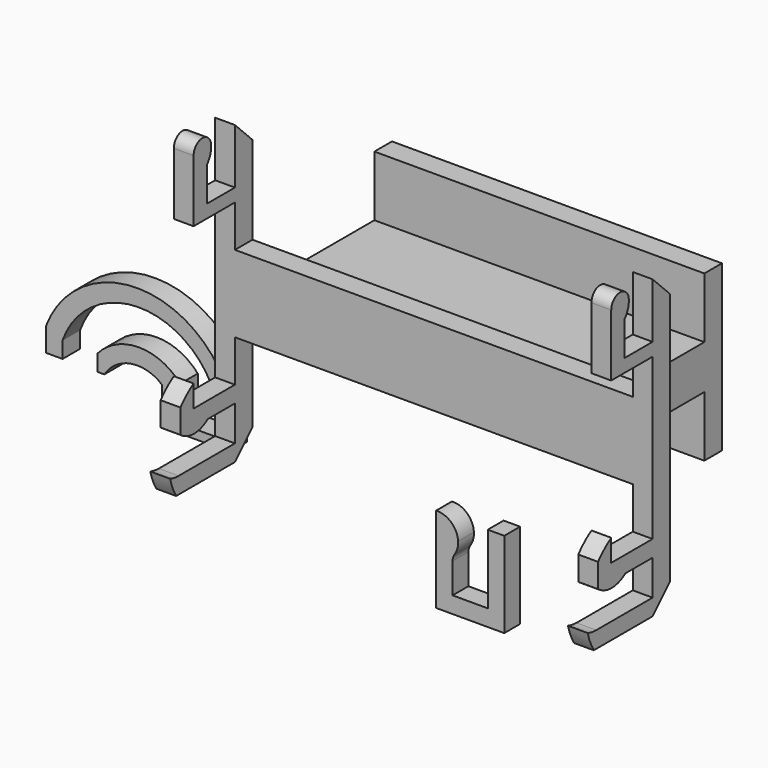
from build123d import *

# Parameters (mm, degrees)
F1_DEPTH  = 5.08
F2_W      = 3.81
F2_H      = 3.81
F2_H_2    = 16.002
F3_DEPTH  = 4.572
F4_R      = 2.54
F6_DEPTH  = 8.89
F5_W      = 12.065
F5_H      = 25.4
F7_W      = 76.2508
F7_H      = 38.1
F8_DEPTH  = 5.08
F11_DEPTH = 50.546
F12_W     = 12.4206
F12_H     = 25.4
F13_DEPTH = 25.4
F14_W     = 91.948
F14_H     = 25.4
F15_DEPTH = 25.4
F16_W     = 8.128
F16_H     = 3.0225940797
F16_W_2   = 3.81
F17_DEPTH = 50.546
F18_R     = 2.54
F19_SIZE  = 5.07999
F20_SIZE  = 5.07999
F22_DEPTH = 25.4
F23_SIZE  = 5.08
F24_SIZE  = 5.08
F25_DEPTH = 57.15
F26_R     = 7.62
F27_R     = 7.62
F29_DEPTH = 101.092


# Not quite as in the source:
# - a fillet or chamfer is up to 0.001 mm smaller than in the source, because OpenCascade refuses the exact size
# - a feature names something its author has since deleted; it is built from what else it names


with BuildPart() as f1:
    # F0 (on Front) → F1 (new body)
    with BuildSketch(Plane.XZ):
        with BuildLine():
            Line((-13.6702175791, 3.3680211509), (-13.6702175791, 11.4960211509))
            ThreePointArc((-13.6702175791, 11.4960211509), (-23.1952175791, 15.7957607383), (-32.7202175791, 11.4960211509))
            Line((-32.7202175791, 11.4960211509), (-32.7202175791, 7.6860211509))
            Line((-32.7202175791, 7.6860211509), (-31.1910058421, 7.6860211509))
            ThreePointArc((-31.1910058421, 7.6860211509), (-25.0379678472, 11.8650180854), (-17.8627536235, 9.9053771004))
            Line((-17.8627536235, 9.9053771004), (-17.8627536235, 1.3360211509))
            Line((-17.8627536235, 1.3360211509), (-2.2494181128, 1.3360211509))
            Line((-2.2494181128, 1.3360211509), (-2.2494181128, 12.5290875188))
            ThreePointArc((-2.2494181128, 12.5290875188), (-23.214575579, 27.7308374634), (-44.6582175791, 13.2118413985))
            Line((-44.6582175791, 13.2118413985), (-44.6582175791, 7.6860211509))
            Line((-44.6582175791, 7.6860211509), (-40.8482175791, 7.6860211509))
            Line((-40.8482175791, 7.6860211509), (-40.8482175791, 11.4960211509))
            ThreePointArc((-40.8482175791, 11.4960211509), (-23.3892785102, 23.9227565337), (-5.6768820684, 11.8600322155))
            Line((-5.6768820684, 11.8600322155), (-5.6768820684, 3.3680211509))
            Line((-5.6768820684, 3.3680211509), (-13.6702175791, 3.3680211509))
        make_face()
    extrude(amount=F1_DEPTH)


with BuildPart() as f3:
    # F2 (on Front) → F3 (new body)
    with BuildSketch(Plane.XZ):
        with Locations((46.9784255706, -13.335)):
            Rectangle(F2_W, F2_H)
        Polygon((60.8214255706, -15.24), (60.8214255706, -11.43), (57.0114255706, -11.43), (48.8834255706, -11.43), (48.8834255706, -15.24), align=None)
        with BuildLine():
            Line((45.0734255706, -11.43), (48.8834255706, -11.43))
            Line((48.8834255706, -11.43), (48.8834255706, -3.556))
            ThreePointArc((48.8834255706, -3.556), (49.8785151524, -1.9066034221), (50.1534255706, 0))
            ThreePointArc((50.1534255706, 0), (48.5549154183, 3.3320998308), (45.0734255706, 4.572))
            Line((45.0734255706, 4.572), (45.0734255706, -11.43))
        make_face()
        with Locations((58.9164255706, -3.429)):
            Rectangle(F2_W, F2_H_2)
    extrude(amount=F3_DEPTH)

    # F4
    f4_edges = [f3.edges().sort_by_distance(p)[0] for p in [
        (48.883426, -2.286, -3.556),
    ]]
    fillet(f4_edges, radius=F4_R)


with BuildPart() as f6:
    # F5 (on Front) → F6 (new body)
    with BuildSketch(Plane.XZ):
        with BuildLine():
            Line((64.2612756615, 64.0052915247), (64.2612756615, 56.3852915247))
            ThreePointArc((64.2612756615, 56.3852915247), (65.1168167537, 54.3198326169), (67.1822756615, 53.4642915247))
            Line((67.1822756615, 53.4642915247), (84.0748242118, 53.4642915247))
            Line((84.0748242118, 53.4642915247), (88.6452756615, 58.0347429745))
            Line((88.6452756615, 58.0347429745), (88.6452756615, 62.3558400749))
            Line((88.6452756615, 62.3558400749), (84.0748242118, 66.9262915247))
            Line((84.0748242118, 66.9262915247), (67.1822756615, 66.9262915247))
            ThreePointArc((67.1822756615, 66.9262915247), (65.1168167537, 66.0707504326), (64.2612756615, 64.0052915247))
        make_face()
        with BuildLine():
            Line((83.5487729875, 54.7342915247), (67.1822756615, 54.7342915247))
            ThreePointArc((67.1822756615, 54.7342915247), (66.0148423658, 55.217858229), (65.5312756615, 56.3852915247))
            Line((65.5312756615, 56.3852915247), (65.5312756615, 64.0052915247))
            ThreePointArc((65.5312756615, 64.0052915247), (66.0148423658, 65.1727248204), (67.1822756615, 65.6562915247))
            Line((67.1822756615, 65.6562915247), (83.5487729875, 65.6562915247))
            Line((83.5487729875, 65.6562915247), (87.3752756615, 61.8297888507))
            Line((87.3752756615, 61.8297888507), (87.3752756615, 58.5607941987))
            Line((87.3752756615, 58.5607941987), (83.5487729875, 54.7342915247))
        make_face(mode=Mode.SUBTRACT)
    extrude(amount=F6_DEPTH)



with BuildPart() as f6b:
    # F5 (on Front) → F6, piece 2 (new body)
    with BuildSketch(Plane.XZ):
        with Locations((53.9104570084, 60.1952915247)):
            Rectangle(F5_W, F5_H)
    extrude(amount=F6_DEPTH)


with BuildPart() as f6c:
    # F5 (on Front) → F6, piece 3 (new body)
    with BuildSketch(Plane.XZ):
        with Locations((98.9955507601, 60.1952915247)):
            Rectangle(F5_W, F5_H)
    extrude(amount=F6_DEPTH)


with BuildPart() as f6_1:
    add(f6.part)

    add(f6b.part)  # F8 merges F6b

    add(f6c.part)  # F8 merges F6c
    # F7 (on face) → F8 (join)
    with BuildSketch(Plane.XZ.offset(8.89)):
        with Locations((76.4530038843, 60.1952915247)):
            Rectangle(F7_W, F7_H)
        Polygon((59.9429570084, 47.4952915247), (47.8779570084, 47.4952915247), (47.8779570084, 72.8952915247), (59.9429570084, 72.8952915247), (59.9429570084, 67.5330780989), (76.4530038843, 60.1952915247), (59.9429570084, 52.8575049505), align=None, mode=Mode.SUBTRACT)
        Polygon((59.9429570084, 72.8952915247), (47.8779570084, 72.8952915247), (59.9429570084, 67.5330780989), align=None)
        Polygon((59.9429570084, 67.5330780989), (59.9429570084, 52.8575049505), (76.4530038843, 60.1952915247), align=None)
        Polygon((47.8779570084, 72.8952915247), (47.8779570084, 47.4952915247), (59.9429570084, 52.8575049505), (59.9429570084, 67.5330780989), align=None)
        Polygon((59.9429570084, 52.8575049505), (47.8779570084, 47.4952915247), (59.9429570084, 47.4952915247), align=None)
    extrude(amount=F8_DEPTH)

    # F10 (on offset) → F11 (join, symmetric)
    with BuildSketch(Plane(origin=(76.4530038843, 0, 0), x_dir=(0, -1, 0), z_dir=(-1, 0, 0))):
        Polygon((39.37, 65.2752915247), (13.97, 65.2752915247), (13.97, 60.1952915247), (44.45, 60.1952915247), (44.45, 94.4852915247), (39.37, 94.4852915247), align=None)
        Polygon((44.45, 60.1952915247), (13.97, 60.1952915247), (13.97, 55.1152915247), (39.37, 55.1152915247), (39.37, 25.9052915247), (44.45, 25.9052915247), align=None)
    extrude(amount=F11_DEPTH, both=True)

    # F12 (on face) → F13 (cut)
    with BuildSketch(Plane.XY.offset(65.2752915247)):
        with Locations((32.1173038843, -26.67)):
            Rectangle(F12_W, F12_H)
        with Locations((120.7887038843, -26.67)):
            Rectangle(F12_W, F12_H)
    extrude(amount=-F13_DEPTH, mode=Mode.SUBTRACT)

    # F14 (on face) → F15 (cut)
    with BuildSketch(Plane.XZ.offset(44.45)):
        with Locations((76.4530038843, 81.7852915247)):
            Rectangle(F14_W, F14_H)
        with Locations((76.4530038843, 38.6052915247)):
            Rectangle(F14_W, F14_H)
    extrude(amount=-F15_DEPTH, mode=Mode.SUBTRACT)

    # F16 (on offset) → F17 (join, symmetric)
    with BuildSketch(Plane(origin=(76.4530038843, 0, 0), x_dir=(0, -1, 0), z_dir=(-1, 0, 0))):
        with Locations((48.514, 80.2485885645)):
            Rectangle(F16_W, F16_H)
        Polygon((68.326, 29.7152915247), (44.45, 29.7152915247), (44.45, 25.9052915247), (72.136, 25.9052915247), (72.136, 49.2732915247), (68.326, 49.2732915247), align=None)
        with BuildLine():
            Line((56.388, 41.6532915247), (44.45, 41.6532915247))
            Line((44.45, 41.6532915247), (44.45, 37.8432915247))
            Line((44.45, 37.8432915247), (52.324, 37.8432915247))
            ThreePointArc((52.324, 37.8432915247), (56.261, 36.4755130172), (60.198, 37.8432915247))
            Line((60.198, 37.8432915247), (60.198, 49.2732915247))
            Line((60.198, 49.2732915247), (56.388, 49.2732915247))
            Line((56.388, 49.2732915247), (56.388, 41.6532915247))
        make_face()
        with Locations((54.483, 80.2485885645)):
            Rectangle(F16_W_2, F16_H)
        with BuildLine():
            Line((52.578, 89.6338856044), (52.578, 81.7598856044))
            Line((52.578, 81.7598856044), (56.388, 81.7598856044))
            Line((56.388, 81.7598856044), (56.388, 97.7618856044))
            ThreePointArc((56.388, 97.7618856044), (52.9065101523, 96.5219854351), (51.308, 93.1898856044))
            ThreePointArc((51.308, 93.1898856044), (51.5829104182, 91.2832821823), (52.578, 89.6338856044))
        make_face()
    extrude(amount=F17_DEPTH, both=True)

    # F18
    f18_edges = [f6_1.edges().sort_by_distance(p)[0] for p in [
        (76.453004, -56.388, 97.761886),
    ]]
    fillet(f18_edges, radius=F18_R)

    # F19 (size 5.08 in the source; OpenCascade refuses exactly that, so slightly less here)
    f19_edges = [f6_1.edges().sort_by_distance(p)[0] for p in [
        (28.193004, -39.37, 94.485292),
    ]]
    chamfer(f19_edges, length=F19_SIZE)

    # F20 (size 5.08 in the source; OpenCascade refuses exactly that, so slightly less here)
    f20_edges = [f6_1.edges().sort_by_distance(p)[0] for p in [
        (124.713004, -39.37, 94.485292),
    ]]
    chamfer(f20_edges, length=F20_SIZE)

    # F21 (on face) → F22 (cut)
    with BuildSketch(Plane(origin=(0, 0, 78.7372915247), x_dir=(1, 0, 0), z_dir=(0, 0, -1))):
        Polygon((30.4790038843, 56.388), (30.4790038843, 44.45), (122.4270038843, 44.45), (122.4270038843, 72.136), (30.4790038843, 72.136), align=None)
    extrude(amount=-F22_DEPTH, mode=Mode.SUBTRACT)

    # F23
    f23_edges = [f6_1.edges().sort_by_distance(p)[0] for p in [
        (28.193004, -39.37, 25.905292),
    ]]
    chamfer(f23_edges, length=F23_SIZE)

    # F24
    f24_edges = [f6_1.edges().sort_by_distance(p)[0] for p in [
        (124.713004, -39.37, 25.905292),
    ]]
    chamfer(f24_edges, length=F24_SIZE)

    # F21 (on face) → F25 (cut, symmetric)
    with BuildSketch(Plane(origin=(0, 0, 78.7372915247), x_dir=(1, 0, 0), z_dir=(0, 0, -1))):
        Polygon((30.4790038843, 56.388), (30.4790038843, 44.45), (122.4270038843, 44.45), (122.4270038843, 72.136), (30.4790038843, 72.136), align=None)
    extrude(amount=F25_DEPTH, both=True, mode=Mode.SUBTRACT)

    # F26
    f26_edges = [f6_1.edges().sort_by_distance(p)[0] for p in [
        (124.713004, -72.136, 25.905292),
        (124.713004, -68.326, 29.715292),
    ]]
    fillet(f26_edges, radius=F26_R)

    # F27
    f27_edges = [f6_1.edges().sort_by_distance(p)[0] for p in [
        (28.193004, -72.136, 25.905292),
        (28.193004, -68.326, 29.715292),
    ]]
    fillet(f27_edges, radius=F27_R)

    # F28 (on face) → F29 (cut, through all)
    with BuildSketch(Plane.YZ.offset(126.9990038843)):
        with BuildLine():
            ThreePointArc((-60.598748991, 24.6616829248), (-63.0615335267, 37.892157408), (-54.0813514617, 47.9154848394))
            Line((-54.0813514617, 47.9154848394), (-60.1272594347, 63.0867996139))
            ThreePointArc((-60.1272594347, 63.0867996139), (-78.4719237933, 43.3532709658), (-74.9058635737, 16.6470530035))
            Line((-74.9058635737, 16.6470530035), (-60.598748991, 24.6616829248))
        make_face()
    extrude(amount=-F29_DEPTH, mode=Mode.SUBTRACT)


solid = Compound([f1.part, f3.part, f6_1.part])
